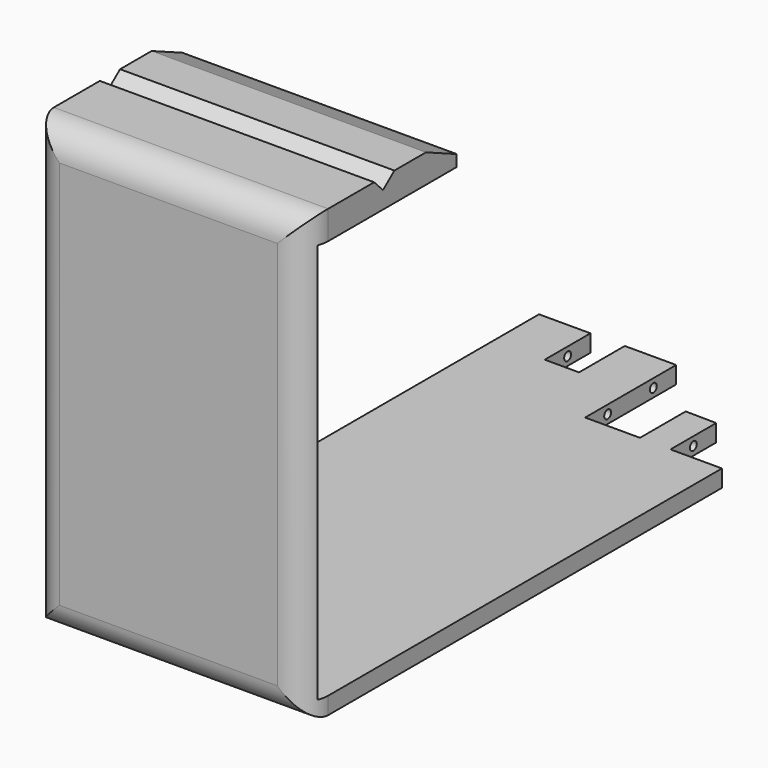
from build123d import *

# Parameters (mm, degrees)
F1_DEPTH      = 3
F3_DEPTH      = 48
F4_T1_DEPTH   = 73.0048285071
F4_T3_DEPTH   = 103.0048285071
F5_R          = 0.75
F6_DEPTH      = 39.001
F7_R          = 0.75
F8_DEPTH      = 9.001
F8_DEPTH_BACK = 39.001


# Not quite as in the source:
# - a fillet or chamfer that OpenCascade refuses, or shapes differently, is made with other operations: its cross-section is extruded or revolved along the edge and cut away or added


with BuildPart() as f1:
    # F0 (on Top) → F1 (new body)
    with BuildSketch(Plane.XY):
        Polygon((-24, 0), (0, 0), (24, 0), (24, 88), (15, 88), (15, 98), (9.6, 98.0832448602), (9.6, 88.0832448602), (0, 88.0832448602), (0, 108), (-9, 108), (-9, 98), (-15, 98), (-15, 108), (-24, 108), align=None)
    extrude(amount=F1_DEPTH)

    # F2 (on face) → F3 (join)
    with BuildSketch(Plane.YZ.offset(24)):
        Polygon((-3.0602848184, 0), (0, 0), (0, 73), (30, 73), (29.9925141591, 74.9999859905), (23.2637450099, 78), (16.367437318, 78), (13.8705000281, 76), (11.9397151816, 78), (-3.0602848184, 78), align=None)
    extrude(amount=-F3_DEPTH)

    # F4: fillet of radius 5 on 6 edges, made by hand

    # F4_s2 → F4_t1 (cut)
    with BuildSketch(Plane.YZ.offset(-36.5024142536)):
        with BuildLine():
            ThreePointArc((-3.0606848184, 72.9990343146), (-1.5958187243, 76.5355339059), (1.9406808671, 78.0004))
            Line((1.9406808671, 78.0004), (1.9406808671, 78.5005365685))
            ThreePointArc((1.9406808671, 78.5005365685), (-0.5598019756, 78.5001365685), (-3.0602848184, 78.5001365685))
            Line((-3.0602848184, 78.5001365685), (-3.5604213869, 78))
            ThreePointArc((-3.5604213869, 78), (-3.5604213869, 75.4995171573), (-3.5608213869, 72.9990343146))
            Line((-3.5608213869, 72.9990343146), (-3.0606848184, 72.9990343146))
        make_face()
        with BuildLine():
            ThreePointArc((1.9406808671, -0.0004), (-1.5958187243, 1.4644660941), (-3.0606848184, 5.0009656854))
            Line((-3.0606848184, 5.0009656854), (-3.5608213869, 5.0009656854))
            ThreePointArc((-3.5608213869, 5.0009656854), (-3.5604213869, 2.5004828427), (-3.5604213869, 0))
            Line((-3.5604213869, 0), (-3.0602848184, -0.5001365685))
            ThreePointArc((-3.0602848184, -0.5001365685), (-0.5598019756, -0.5001365685), (1.9406808671, -0.5005365685))
            Line((1.9406808671, -0.5005365685), (1.9406808671, -0.0004))
        make_face()
    extrude(amount=F4_T1_DEPTH, mode=Mode.SUBTRACT)

    # F4_s4 → F4_t3 (cut)
    with BuildSketch(Plane.XY.offset(-12.5024142536)):
        with BuildLine():
            ThreePointArc((18.9990343146, -3.0606848184), (22.5355339059, -1.5958187243), (24.0004, 1.9406808671))
            Line((24.0004, 1.9406808671), (24.5005365685, 1.9406808671))
            ThreePointArc((24.5005365685, 1.9406808671), (24.5001365685, -0.5598019756), (24.5001365685, -3.0602848184))
            Line((24.5001365685, -3.0602848184), (24, -3.5604213869))
            ThreePointArc((24, -3.5604213869), (21.4995171573, -3.5604213869), (18.9990343146, -3.5608213869))
            Line((18.9990343146, -3.5608213869), (18.9990343146, -3.0606848184))
        make_face()
        with BuildLine():
            ThreePointArc((-18.9990343146, -3.0606848184), (-22.5355339059, -1.5958187243), (-24.0004, 1.9406808671))
            Line((-24.0004, 1.9406808671), (-24.5005365685, 1.9406808671))
            ThreePointArc((-24.5005365685, 1.9406808671), (-24.5001365685, -0.5598019756), (-24.5001365685, -3.0602848184))
            Line((-24.5001365685, -3.0602848184), (-24, -3.5604213869))
            ThreePointArc((-24, -3.5604213869), (-21.4995171573, -3.5604213869), (-18.9990343146, -3.5608213869))
            Line((-18.9990343146, -3.5608213869), (-18.9990343146, -3.0606848184))
        make_face()
    extrude(amount=F4_T3_DEPTH, mode=Mode.SUBTRACT)

    # F5 (on face) → F6 (cut, through all)
    with BuildSketch(Plane.YZ.offset(15)):
        with Locations((93, 1.5)):
            Circle(F5_R)
    extrude(amount=-F6_DEPTH, mode=Mode.SUBTRACT)

    # F7 (on face) → F8 (cut, two sides)
    with BuildSketch(Plane.YZ.offset(-15)) as f8_sk:
        with Locations((103, 1.5)):
            Circle(F7_R)
    extrude(amount=-F8_DEPTH, mode=Mode.SUBTRACT)
    extrude(f8_sk.sketch, amount=F8_DEPTH_BACK, mode=Mode.SUBTRACT)


solid = f1.part
